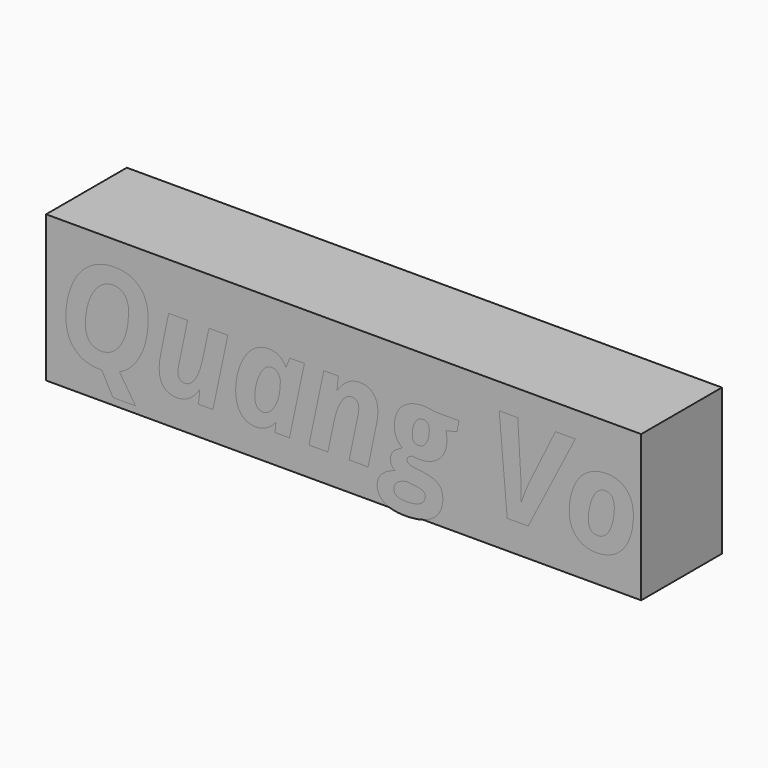
from build123d import *

# Parameters (mm, degrees)
F1_W         = 149.7696116567
F1_H         = 36.8254799396
F2_DEPTH     = 25.4
F0_TEXT_SIZE = 32.4279354471
F3_DEPTH     = 25.4


# Not quite as in the source:
# - Text() gives the source's letters only with a copy of the font that has no kerning and outlines rounded to 1/6400 em; it was checked with that copy


with BuildPart() as f2:
    # F1 (on Front) → F2 (new body)
    with BuildSketch(Plane.XZ):
        with Locations((0.2847351134, 3.8913516328)):
            Rectangle(F1_W, F1_H)
    extrude(amount=F2_DEPTH)


with BuildPart() as f3:
    # F0 (on Front) → F3 (new body)
    with BuildSketch(Plane.XZ):
        with Locations((-71.5629197657, -7.3081506416)):
            Text('Quang Vo', F0_TEXT_SIZE, font='Open Sans', font_style=FontStyle.BOLDITALIC, text_align=(TextAlign.LEFT, TextAlign.BOTTOM))
    extrude(amount=F3_DEPTH)


solid = Compound([f2.part, f3.part])
